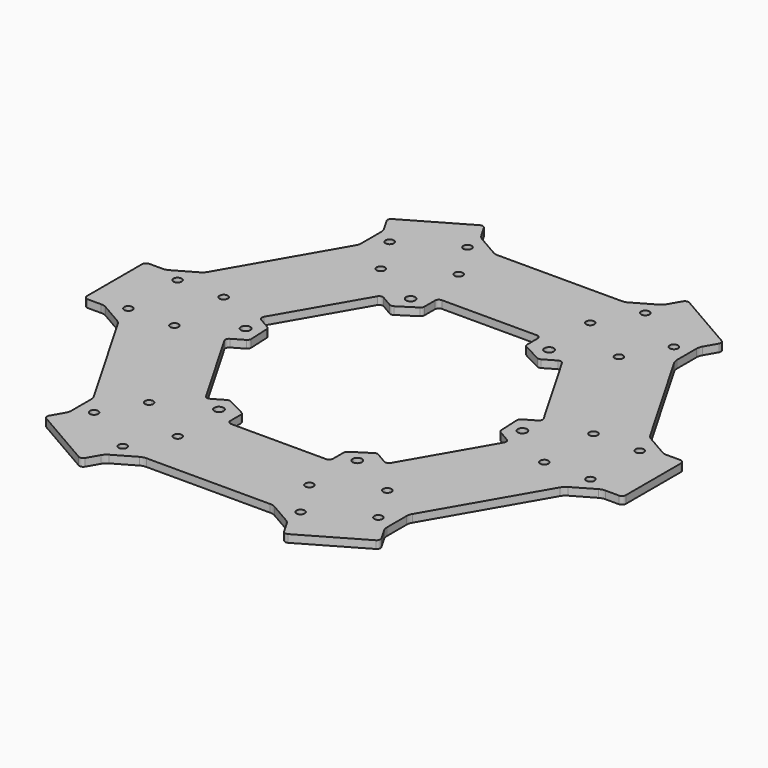
from build123d import *

# Parameters (mm, degrees)
F1_DEPTH        = 2
F3_D            = 2.4
F4_R            = 1
F5_R            = 3
F7_D            = 2.15
F7_COPIES_COUNT = 6


# Not quite as in the source:
# - a pattern or mirror of a feature is missing from the dataset's text; its kind, count and spacing are read off the source's solid


with BuildPart() as f1:
    # F0 (on Top) → F1 (new body)
    with BuildSketch(Plane.XY):
        Polygon((16.9, 57.1576766498), (-16.9, 57.1576766498), (-23.7294919243, 61.1006856507), (-26.393684127, 65.7152019068), (-43.7141922027, 55.7152019068), (-41.05, 51.1006856507), (-41.05, 43.2146676488), (-57.95, 13.9430090009), (-64.7794919243, 10), (-70.1078763296, 10), (-70.1078763296, -10), (-64.7794919243, -10), (-57.95, -13.9430090009), (-41.05, -43.2146676488), (-41.05, -51.1006856507), (-43.7141922027, -55.7152019068), (-26.393684127, -65.7152019068), (-23.7294919243, -61.1006856507), (-16.9, -57.1576766498), (16.9, -57.1576766498), (23.7294919243, -61.1006856507), (26.393684127, -65.7152019068), (43.7141922027, -55.7152019068), (41.05, -51.1006856507), (41.05, -43.2146676488), (57.95, -13.9430090009), (64.7794919243, -10), (70.1078763296, -10), (70.1078763296, 10), (64.7794919243, 10), (57.95, 13.9430090009), (41.05, 43.2146676488), (41.05, 51.1006856507), (43.7141922027, 55.7152019068), (26.393684127, 65.7152019068), (23.7294919243, 61.1006856507), align=None)
        Polygon((-23.4683549509, 28.6336491577), (-20, 34.6410161514), (-13.6476270854, 34.6410161514), (13.0632900982, 34.6410161514), (20, 34.6410161514), (23.1761864573, 29.1396998331), (36.5316450491, 6.0073669937), (40, 0), (36.8238135427, -5.5013163183), (23.4683549509, -28.6336491577), (20, -34.6410161514), (13.6476270854, -34.6410161514), (-13.0632900982, -34.6410161514), (-20, -34.6410161514), (-23.1761864573, -29.1396998331), (-36.5316450491, -6.0073669937), (-40, 0), (-36.8238135427, 5.5013163183), align=None, mode=Mode.SUBTRACT)
        Polygon((-13.6476270854, 34.6410161514), (-20, 34.6410161514), (-23.4683549509, 28.6336491577), (-19.138227932, 26.1336491577), (-13.6476270854, 29.6410161514), align=None)
        Polygon((-32.4936865238, 3.0013163183), (-36.8238135427, 5.5013163183), (-40, 0), (-36.5316450491, -6.0073669937), (-32.2015180302, -3.5073669937), align=None)
        Polygon((20, 34.6410161514), (13.0632900982, 34.6410161514), (13.0632900982, 29.6410161514), (18.8460594384, 26.6396998331), (23.1761864573, 29.1396998331), align=None)
        Polygon((40, 0), (36.5316450491, 6.0073669937), (32.2015180302, 3.5073669937), (32.4936865238, -3.0013163183), (36.8238135427, -5.5013163183), align=None)
        Polygon((20, -34.6410161514), (23.4683549509, -28.6336491577), (19.138227932, -26.1336491577), (13.6476270854, -29.6410161514), (13.6476270854, -34.6410161514), align=None)
        Polygon((-18.8460594384, -26.6396998331), (-23.1761864573, -29.1396998331), (-20, -34.6410161514), (-13.0632900982, -34.6410161514), (-13.0632900982, -29.6410161514), align=None)
    extrude(amount=F1_DEPTH)

    # F3 (through all)
    with Locations(Plane(origin=(0, 0, 0), x_dir=(1, 0, 0), z_dir=(0, 0, -1))):
        with Locations((-36, 0), (-18, -31.1769145362), (18, -31.1769145362), (36, 0), (18, 31.1769145362), (-18, 31.1769145362)):
            Hole(F3_D / 2)

    # F4
    f4_edges = [f1.edges().sort_by_distance(p)[0] for p in [
        (-26.393684, -65.715202, 1),
        (-43.714192, -55.715202, 1),
        (26.393684, -65.715202, 1),
        (43.714192, -55.715202, 1),
        (70.107876, -10, 1),
        (70.107876, 10, 1),
        (26.393684, 65.715202, 1),
        (43.714192, 55.715202, 1),
        (-26.393684, 65.715202, 1),
        (-43.714192, 55.715202, 1),
        (-70.107876, 10, 1),
        (-70.107876, -10, 1),
        (32.201518, 3.507367, 1),
        (32.493687, -3.001316, 1),
        (13.647627, -29.641016, 1),
        (19.138228, -26.133649, 1),
        (-18.846059, -26.6397, 1),
        (-13.06329, -29.641016, 1),
        (-32.493687, 3.001316, 1),
        (-32.201518, -3.507367, 1),
        (-19.138228, 26.133649, 1),
        (-13.647627, 29.641016, 1),
        (13.06329, 29.641016, 1),
        (18.846059, 26.6397, 1),
        (23.176186, 29.1397, 1),
        (13.06329, 34.641016, 1),
        (36.823814, -5.501316, 1),
        (36.531645, 6.007367, 1),
        (23.468355, -28.633649, 1),
        (13.647627, -34.641016, 1),
        (-13.06329, -34.641016, 1),
        (-36.823814, 5.501316, 1),
        (-36.531645, -6.007367, 1),
        (-23.176186, -29.1397, 1),
        (-13.647627, 34.641016, 1),
        (-23.468355, 28.633649, 1),
    ]]
    fillet(f4_edges, radius=F4_R)

    # F5
    f5_edges = [f1.edges().sort_by_distance(p)[0] for p in [
        (-64.779492, -10, 1),
        (-57.95, -13.943009, 1),
        (-41.05, -43.214668, 1),
        (-41.05, -51.100686, 1),
        (-16.9, -57.157677, 1),
        (-23.729492, -61.100686, 1),
        (16.9, -57.157677, 1),
        (23.729492, -61.100686, 1),
        (41.05, -51.100686, 1),
        (41.05, -43.214668, 1),
        (57.95, -13.943009, 1),
        (64.779492, -10, 1),
        (57.95, 13.943009, 1),
        (64.779492, 10, 1),
        (41.05, 51.100686, 1),
        (41.05, 43.214668, 1),
        (23.729492, 61.100686, 1),
        (16.9, 57.157677, 1),
        (-16.9, 57.157677, 1),
        (-23.729492, 61.100686, 1),
        (-41.05, 43.214668, 1),
        (-41.05, 51.100686, 1),
        (-64.779492, 10, 1),
        (-57.95, 13.943009, 1),
    ]]
    fillet(f5_edges, radius=F5_R)

    # F7 (through all)
    with Locations(Plane.XY.offset(2)):
        with Locations((-48.1078763296, 8), (-48.1078763296, -8), (-60.1078763296, -8), (-60.1078763296, 8)):
            f7 = Hole(F7_D / 2)

    # F7_copies: F7 ×6 about axis
    f7_copies_axis = Axis((0, 0, 0), (0, 0, 1))
    for i in range(1, F7_COPIES_COUNT):
        add(f7.rotate(f7_copies_axis, i * 360 / F7_COPIES_COUNT), mode=Mode.SUBTRACT)


solid = f1.part
